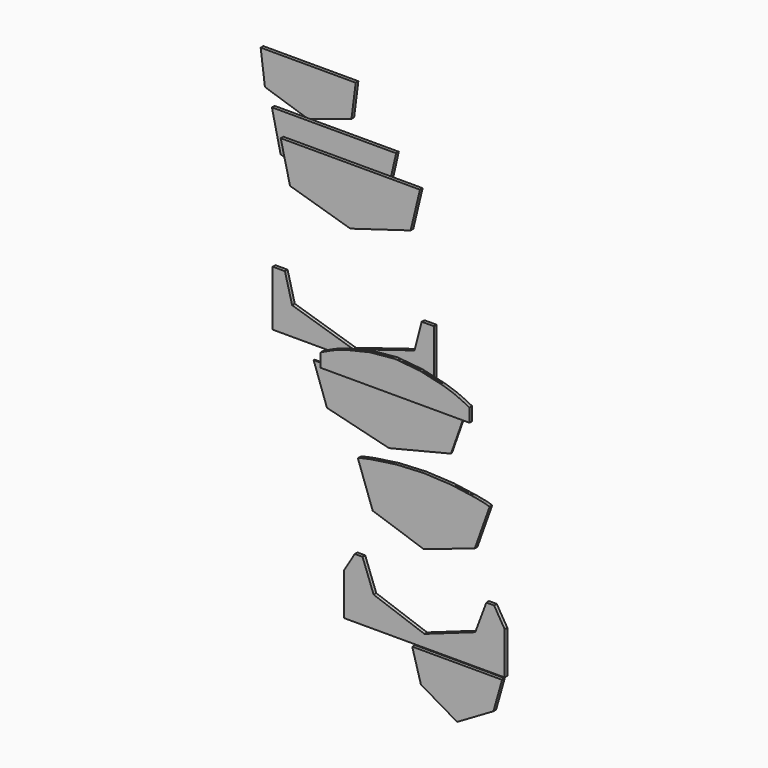
from build123d import *

# Parameters (mm, degrees)
F3_DEPTH  = 6
F6_DEPTH  = 6
F8_DEPTH  = 6
F11_DEPTH = 6
F14_DEPTH = 2
F17_DEPTH = 6
F20_DEPTH = 6
F23_DEPTH = 6
F26_DEPTH = 6


# Not quite as in the source:
# - the dataset's text gives a spline's control points without its knots; the knots are read off the source's solid


with BuildPart() as f3:
    # F2 (on offset) → F3 (new body, symmetric)
    with BuildSketch(Plane.XZ.offset(-50)):
        Polygon((-1881.5177679062, 681.6917657852), (-1663.2950305939, 746.8433380127), (-1629.4765472412, 887.7972960472), (-1881.5177679062, 887.7972960472), align=None)
        Polygon((-2099.7405052185, 746.8433380127), (-1881.5177679062, 681.6917657852), (-1881.5177679062, 887.7972960472), (-2133.5589885712, 887.7972960472), align=None)
    extrude(amount=F3_DEPTH, both=True)


with BuildPart() as f6:
    # F5 (on offset) → F6 (new body, symmetric)
    with BuildSketch(Plane.XZ.offset(-345)):
        Polygon((-2176.5863895416, 581.7740559578), (-1983.3632707596, 639.4465565681), (-1951.8201351166, 779.1160345078), (-2176.5863895416, 779.1160345078), align=None)
        Polygon((-2369.8095083237, 639.4465565681), (-2176.5863895416, 581.7740559578), (-2176.5863895416, 779.1160345078), (-2401.3526439667, 779.1160345078), align=None)
    extrude(amount=F6_DEPTH, both=True)


with BuildPart() as f8:
    # F7 (on Front) → F8 (new body, symmetric)
    with BuildSketch(Plane.XZ):
        Polygon((-1583.1931829453, 502.4157166481), (-1609.2249155045, 402.4670124054), (-1830.6815624237, 334.1079950333), (-2052.138209343, 402.4670124054), (-2078.1699419022, 502.4157166481), (-2122.403383255, 502.4157166481), (-2122.403383255, 301.7150759697), (-1830.6815624237, 301.7150759697), (-1538.9597415924, 301.7150759697), (-1538.9597415924, 502.4157166481), align=None)
    extrude(amount=F8_DEPTH, both=True)


with BuildPart() as f11:
    # F10 (on offset) → F11 (new body, symmetric)
    with BuildSketch(Plane.XZ.offset(-800)):
        Polygon((-2477.391242981, 532.4255824089), (-2462.0735645294, 652.8984308243), (-2634.0358257294, 652.8984308243), (-2634.0358257294, 481.3759326935), align=None)
        Polygon((-2634.0358257294, 481.3759326935), (-2634.0358257294, 652.8984308243), (-2805.9980869293, 652.8984308243), (-2790.6804084778, 532.4255824089), align=None)
    extrude(amount=F11_DEPTH, both=True)


with BuildPart() as f14:
    # F13 (on offset) → F14 (new body, symmetric)
    with BuildSketch(Plane.XZ.offset(630)):
        Polygon((-928.0948638916, 670.2681183815), (-1200.793504715, 670.2681183815), (-1473.4921455383, 670.2681183815), (-1425.3154397011, 533.9187979698), (-1200.793504715, 478.4700572491), (-976.2715697289, 533.9187979698), align=None)
    extrude(amount=F14_DEPTH, both=True)


with BuildPart() as f17:
    # F16 (on offset) → F17 (new body, symmetric)
    with BuildSketch(Plane.XZ.offset(740)):
        with BuildLine():
            add(Edge.make_bspline(
                [(-1088.1509780884, 845.8876609802), (-1064.8640734247, 844.5303544338), (-1019.6574488416, 841.8954294243), (-960.6351334614, 830.547216212), (-902.7649512722, 815.3018401586), (-861.6273766032, 800.2954708729), (-832.8945184556, 785.7678831175), (-818.1775808334, 778.3268690109)],
                knots=[0, 0, 0, 0, 0.2219482822, 0.4308658801, 0.6365369525, 0.8138346359, 1, 1, 1, 1], degree=3))
            Line((-1088.1509780884, 845.8876609802), (-1088.1509780884, 729.9741506577))
            Line((-1088.1509780884, 729.9741506577), (-818.1775808334, 729.9741506577))
            Line((-818.1775808334, 729.9741506577), (-818.1775808334, 778.3268690109))
        make_face()
        with BuildLine():
            Line((-1088.1509780884, 729.9741506577), (-1088.1509780884, 845.8876609802))
            add(Edge.make_bspline(
                [(-1088.1509780884, 845.8876609802), (-1111.437882752, 844.5303544338), (-1156.6445073352, 841.8954294243), (-1215.6668227154, 830.547216212), (-1273.5370049046, 815.3018401586), (-1314.6745795736, 800.2954708729), (-1343.4074377211, 785.7678831175), (-1358.1243753433, 778.3268690109)],
                knots=[0, 0, 0, 0, 0.2219482822, 0.4308658801, 0.6365369525, 0.8138346359, 1, 1, 1, 1], degree=3))
            Line((-1358.1243753433, 778.3268690109), (-1358.1243753433, 729.9741506577))
            Line((-1358.1243753433, 729.9741506577), (-1088.1509780884, 729.9741506577))
        make_face()
    extrude(amount=F17_DEPTH, both=True)


with BuildPart() as f20:
    # F19 (on offset) → F20 (new body, symmetric)
    with BuildSketch(Plane.XZ.offset(1255)):
        with BuildLine():
            Line((-756.653636694, 679.2419552803), (-571.8927979469, 616.8168187141))
            Line((-571.8927979469, 616.8168187141), (-387.1319591999, 679.2419552803))
            Line((-387.1319591999, 679.2419552803), (-333.5082530975, 829.2589187622))
            add(Edge.make_bspline(
                [(-571.8927979469, 859.1964244843), (-544.8189911828, 858.6125739832), (-497.0142078125, 857.5816570174), (-451.5883648538, 851.665675284), (-420.1290894013, 847.6665525577), (-389.8967225448, 842.7241954223), (-369.0165662088, 838.4980297127), (-346.6023759232, 834.06862687), (-337.5027643359, 830.7261749767), (-333.5082530975, 829.2589187622)],
                knots=[0, 0, 0, 0, 0.2207569608, 0.3897951544, 0.5312243388, 0.669250984, 0.7873565303, 0.9066546169, 1, 1, 1, 1], degree=3))
            add(Edge.make_bspline(
                [(-571.8927979469, 859.1964244843), (-598.9666047111, 858.6125739832), (-646.7713880814, 857.5816570174), (-692.19723104, 851.665675284), (-723.6565064925, 847.6665525577), (-753.8888733491, 842.7241954223), (-774.7690296851, 838.4980297127), (-797.1832199706, 834.06862687), (-806.282831558, 830.7261749767), (-810.2773427963, 829.2589187622)],
                knots=[0, 0, 0, 0, 0.2207569608, 0.3897951544, 0.5312243388, 0.669250984, 0.7873565303, 0.9066546169, 1, 1, 1, 1], degree=3))
            Line((-810.2773427963, 829.2589187622), (-756.653636694, 679.2419552803))
        make_face()
    extrude(amount=F20_DEPTH, both=True)


with BuildPart() as f23:
    # F22 (on offset) → F23 (new body, symmetric)
    with BuildSketch(Plane.XZ.offset(1270)):
        Polygon((-847.6955890656, 313.3543431759), (-557.308614254, 313.3543431759), (-266.9216394424, 313.3543431759), (-266.9216394424, 466.711461544), (-305.0965666771, 530.3864479065), (-333.261013031, 530.3864479065), (-373.4048306942, 422.9025840759), (-557.308614254, 357.5751781464), (-741.2123978138, 422.9025840759), (-781.356215477, 530.3864479065), (-809.5206618309, 530.3864479065), (-847.6955890656, 466.711461544), align=None)
    extrude(amount=F23_DEPTH, both=True)


with BuildPart() as f26:
    # F25 (on offset) → F26 (new body, symmetric)
    with BuildSketch(Plane.XZ.offset(1860)):
        Polygon((33.1224352121, 509.0515017509), (164.4237786531, 585.6313109398), (195.7399398088, 696.0937380791), (33.1224352121, 696.0937380791), (-129.4950693846, 696.0937380791), (-98.1789082289, 585.6313109398), align=None)
    extrude(amount=F26_DEPTH, both=True)


solid = Compound([f3.part, f6.part, f8.part, f11.part, f14.part, f17.part, f20.part, f23.part, f26.part])
